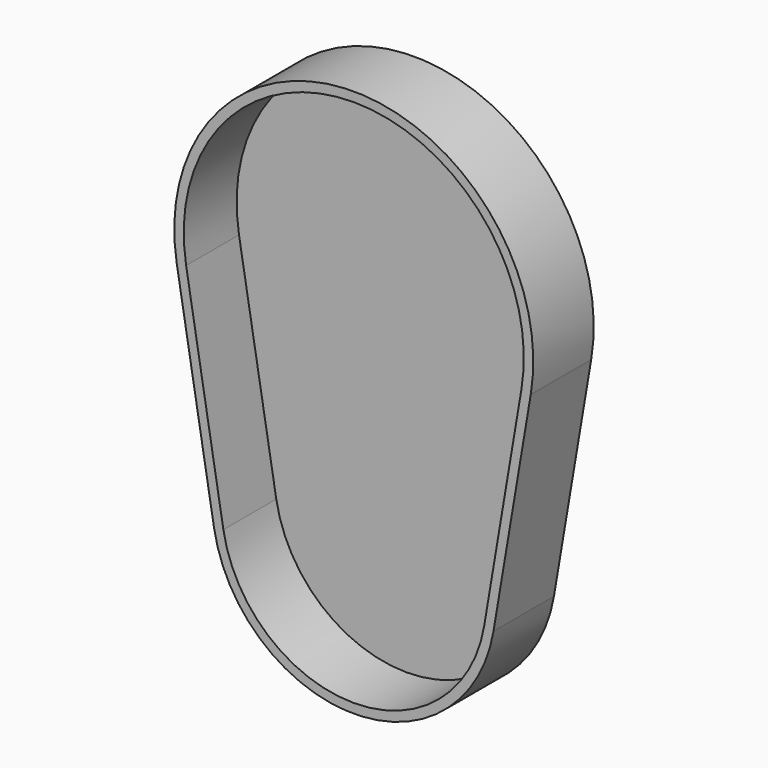
from build123d import *

# Parameters (mm, degrees)
F1_DEPTH = 25.4
F2_T     = -3.175


# Not quite as in the source:
# - ends of sketch curves that miss each other by under 0.0002 mm in the source are joined


with BuildPart() as f1:
    # F0 (on Front) → F1 (new body)
    with BuildSketch(Plane.XZ):
        with BuildLine():
            ThreePointArc((-46.9588833262, -52.3874997171), (0, -92.075), (46.9588833262, -52.3874997171))
            Line((46.9588833262, -52.3874997171), (59.4812628, 21.6958164))
            ThreePointArc((59.4812628, 21.6958164), (0, 92.075), (-59.4812496656, 21.6958186201))
            Line((-59.4812496656, 21.6958186201), (-46.9588833262, -52.3874997171))
        make_face()
    extrude(amount=F1_DEPTH)

    # F2
    f2_openings = [f1.faces().sort_by_distance(p)[0] for p in [
        (4e-06, -25.4, 3.213538),
    ]]
    offset(amount=F2_T, openings=f2_openings, kind=Kind.INTERSECTION)


solid = f1.part
